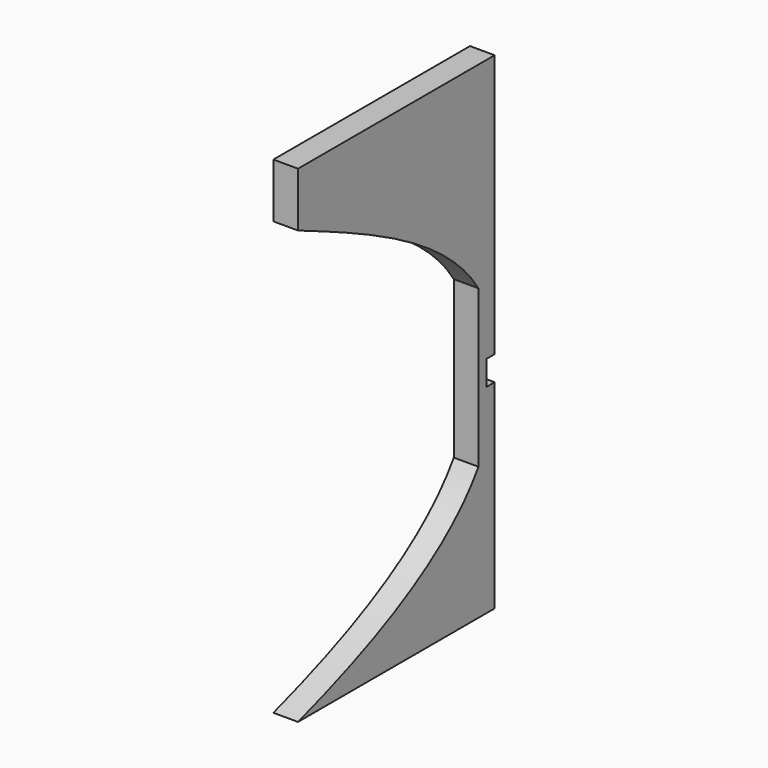
from build123d import *

# Parameters (mm, degrees)
F1_DEPTH = 22


with BuildPart() as f1:
    # F0 (on Right) → F1 (new body)
    with BuildSketch(Plane.YZ):
        with BuildLine():
            Line((109.5, -2.0528280745), (109.5, 217.0326773285))
            Line((109.5, 217.0326773285), (-109.5, 217.0326773285))
            Line((-109.5, 217.0326773285), (-109.5, 168.5))
            add(Edge.make_bspline(
                [(-109.5, 168.5), (-27.7467335676, 133.469891204), (55.4140619779, 97.2245921781), (91.5, 41.4673226715)],
                knots=[0, 0, 0, 0, 0.3625910784, 0.3625910784, 0.3625910784, 0.3625910784], degree=3))
            add(Edge.make_bspline(
                [(91.5, 41.4673226715), (100.2961758102, 27.8761352961), (106.2952978286, 13.1256022765), (109.5, -2.0528280745)],
                knots=[0.3625910784, 0.3625910784, 0.3625910784, 0.3625910784, 0.4509749489, 0.4509749489, 0.4509749489, 0.4509749489], degree=3))
        make_face()
        with BuildLine():
            Line((109.5, -17.5326773285), (109.5, -2.0528280745))
            add(Edge.make_bspline(
                [(91.5, 41.4673226715), (100.2961758102, 27.8761352961), (106.2952978286, 13.1256022765), (109.5, -2.0528280745)],
                knots=[0.3625910784, 0.3625910784, 0.3625910784, 0.3625910784, 0.4509749489, 0.4509749489, 0.4509749489, 0.4509749489], degree=3))
            Line((91.5, 41.4673226715), (91.5, -28.5326773285))
            Line((91.5, -28.5326773285), (91.5, -98.5326773285))
            add(Edge.make_bspline(
                [(109.5, -54.8776239379), (106.2942898962, -70.0854206268), (100.2934101345, -84.8814155055), (91.5, -98.5326773285)],
                knots=[0.5523720652, 0.5523720652, 0.5523720652, 0.5523720652, 0.640815625, 0.640815625, 0.640815625, 0.640815625], degree=3))
            Line((109.5, -54.8776239379), (109.5, -39.5326773285))
            Line((109.5, -39.5326773285), (100.5, -39.5326773285))
            Line((100.5, -39.5326773285), (100.5, -17.5326773285))
            Line((100.5, -17.5326773285), (109.5, -17.5326773285))
        make_face()
        with BuildLine():
            Line((109.5, -217.0326773285), (109.5, -54.8776239379))
            add(Edge.make_bspline(
                [(109.5, -54.8776239379), (106.2942898962, -70.0854206268), (100.2934101345, -84.8814155055), (91.5, -98.5326773285)],
                knots=[0.5523720652, 0.5523720652, 0.5523720652, 0.5523720652, 0.640815625, 0.640815625, 0.640815625, 0.640815625], degree=3))
            add(Edge.make_bspline(
                [(91.5, -98.5326773285), (55.7884622504, -153.9727790026), (-25.9805742583, -190.5326773285), (-109.5, -217.0326773285)],
                knots=[0.640815625, 0.640815625, 0.640815625, 0.640815625, 1, 1, 1, 1], degree=3))
            Line((-109.5, -217.0326773285), (109.5, -217.0326773285))
        make_face()
    extrude(amount=F1_DEPTH)


solid = f1.part
